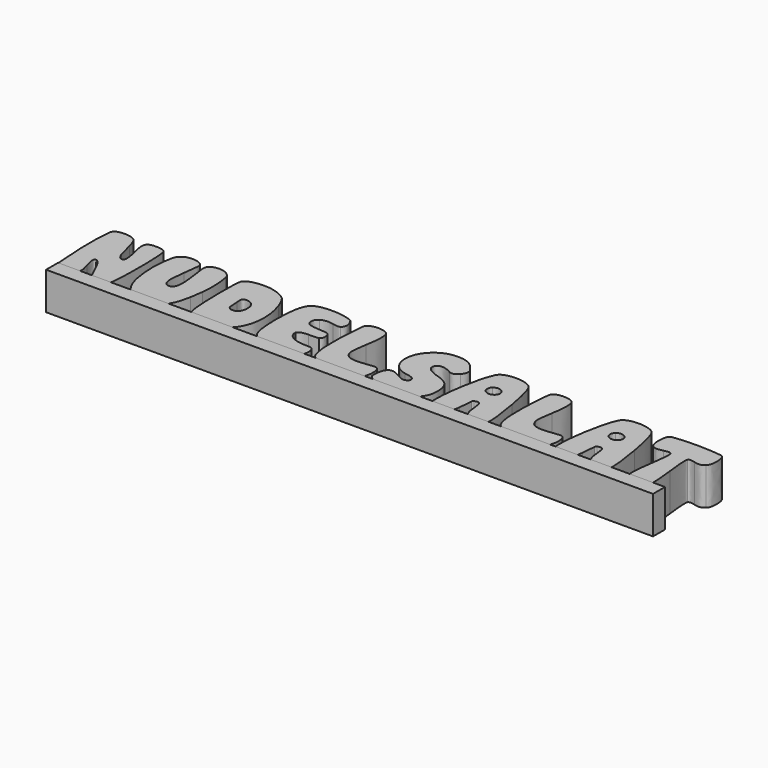
from build123d import *

# Parameters (mm, degrees)
F1_DEPTH = 10
F2_W     = 162
F2_H     = 4
F3_DEPTH = 10


# Not quite as in the source:
# - the dataset's text gives a spline's control points without its knots; the knots are read off the source's solid


with BuildPart() as f1:
    # F0 (on Top) → F1 (new body)
    with BuildSketch(Plane.XY):
        with BuildLine():
            add(Edge.make_bspline(
                [(-78.6229949402, 10.3743381), (-77.2540190734, 10.3743381), (-76.2557894812, 10.0700247503), (-75.628596004, 9.4616875221)],
                knots=[0, 0, 0, 0, 1, 1, 1, 1], degree=3))
            add(Edge.make_bspline(
                [(-81.5318144928, 8.9769327547), (-81.3989493816, 9.9081493719), (-80.4291492678, 10.3743381), (-78.6229949402, 10.3743381)],
                knots=[26, 26, 26, 26, 27, 27, 27, 27], degree=3))
            add(Edge.make_bspline(
                [(-81.3035069281, -8.7327223423), (-81.6841162725, -3.8660267327), (-81.8738407099, 0.0317393925), (-81.8738407099, 2.9597057731), (-81.8738407099, 5.3930535779), (-81.7598318478, 7.3985055723), (-81.5318144928, 8.9769327547)],
                knots=[24, 24, 24, 24, 25, 25, 25, 26, 26, 26, 26], degree=3))
            add(Edge.make_bspline(
                [(-80.1056890901, -9.8449607967), (-80.8094687718, -9.5980868234), (-81.2086445248, -9.2273405489), (-81.3035069281, -8.7327223423)],
                knots=[23, 23, 23, 23, 24, 24, 24, 24], degree=3))
            add(Edge.make_bspline(
                [(-75.6570258517, -8.8183013567), (-75.9804856602, -9.7120953163), (-76.8931362381, -10.158557166), (-78.3946870063, -10.158557166), (-79.0033140749, -10.158557166), (-79.5736482259, -10.0544117431), (-80.1056890901, -9.8449607967)],
                knots=[21, 21, 21, 21, 22, 22, 22, 23, 23, 23, 23], degree=3))
            add(Edge.make_bspline(
                [(-75.9706225903, -5.6100998048), (-75.6097397549, -6.7223382591), (-75.4287179178, -7.5447679435), (-75.4287179178, -8.0768091769), (-75.4287179178, -8.4191256037), (-75.5050139125, -8.6662897867), (-75.6570258517, -8.8183013567)],
                knots=[19, 19, 19, 19, 20, 20, 20, 21, 21, 21, 21], degree=3))
            add(Edge.make_bspline(
                [(-76.0846310832, -2.4871874267), (-76.3700881838, -2.5254803444), (-76.5125268936, -2.7537882783), (-76.5125268936, -3.1718202804), (-76.5125268936, -3.6850048955), (-76.3320854759, -4.4978613505), (-75.9706225903, -5.6100998048)],
                knots=[17, 17, 17, 17, 18, 18, 18, 19, 19, 19, 19], degree=3))
            add(Edge.make_bspline(
                [(-74.2596205065, -4.5405059374), (-74.9253967418, -3.2101135672), (-75.5334437602, -2.5254803444), (-76.0846310832, -2.4871874267)],
                knots=[16, 16, 16, 16, 17, 17, 17, 17], degree=3))
            add(Edge.make_bspline(
                [(-72.463039039, -8.2479672057), (-73.2613909142, -6.5938244481), (-73.8604443843, -5.358294112), (-74.2596205065, -4.5405059374)],
                knots=[15, 15, 15, 15, 16, 16, 16, 16], degree=3))
            add(Edge.make_bspline(
                [(-71.2367920918, -9.5882233842), (-71.9025683272, -9.2650534162), (-72.311027469, -8.8183013567), (-72.463039039, -8.2479672057)],
                knots=[14, 14, 14, 14, 15, 15, 15, 15], degree=3))
            add(Edge.make_bspline(
                [(-67.3297425778, -8.9323102188), (-67.4820447267, -9.6549461496), (-68.1666775804, -10.0161188255), (-69.3830614576, -10.0161188255), (-70.048837693, -10.0161188255), (-70.6664579408, -9.8733902751), (-71.2367920918, -9.5882233842)],
                knots=[12, 12, 12, 12, 13, 13, 13, 14, 14, 14, 14], degree=3))
            add(Edge.make_bspline(
                [(-67.3297425778, 9.0625117691), (-67.0068628195, 7.9404102449), (-66.8449878104, 5.1934657014), (-66.8449878104, 0.8208078788), (-66.8449878104, -4.179623102), (-67.0068628195, -7.4307594506), (-67.3297425778, -8.9323102188)],
                knots=[10, 10, 10, 10, 11, 11, 11, 12, 12, 12, 12], degree=3))
            add(Edge.make_bspline(
                [(-72.2634511625, 9.2049504789), (-72.0542900566, 9.7184249346), (-71.3127978768, 9.9748721372), (-70.0389746231, 9.9748721372), (-68.575136353, 9.9748721372), (-67.6720593738, 9.6705587875), (-67.3297425778, 9.0625117691)],
                knots=[8, 8, 8, 8, 9, 9, 9, 10, 10, 10, 10], degree=3))
            add(Edge.make_bspline(
                [(-71.9495645834, 5.183892472), (-72.311027469, 6.5528679696), (-72.4914688867, 7.5888104292), (-72.4914688867, 8.2925897416), (-72.4914688867, 8.729478362), (-72.4157529423, 9.0337920809), (-72.2634511625, 9.2049504789)],
                knots=[6, 6, 6, 6, 7, 7, 7, 8, 8, 8, 8], degree=3))
            add(Edge.make_bspline(
                [(-71.9211347357, 1.0775452913), (-71.5788183089, 1.1344046174), (-71.4079501206, 1.4668576051), (-71.4079501206, 2.0754846737), (-71.4079501206, 2.7786839359), (-71.588681748, 3.815206815), (-71.9495645834, 5.183892472)],
                knots=[4, 4, 4, 4, 5, 5, 5, 6, 6, 6, 6], degree=3))
            add(Edge.make_bspline(
                [(-73.489698479, 2.8454067013), (-73.03337319, 1.5715834475), (-72.5106153455, 0.9821028377), (-71.9211347357, 1.0775452913)],
                knots=[3, 3, 3, 3, 4, 4, 4, 4], degree=3))
            add(Edge.make_bspline(
                [(-74.5163575497, 6.6953066794), (-73.9651702267, 4.4711199804), (-73.6228537999, 3.1877231281), (-73.489698479, 2.8454067013)],
                knots=[2, 2, 2, 2, 3, 3, 3, 3], degree=3))
            add(Edge.make_bspline(
                [(-75.628596004, 9.4616875221), (-75.2674233281, 9.1002246365), (-74.8966770536, 8.178291039), (-74.5163575497, 6.6953066794)],
                knots=[1, 1, 1, 1, 2, 2, 2, 2], degree=3))
        make_face()
    extrude(amount=F1_DEPTH)


with BuildPart() as f1b:
    # F0 (on Top) → F1, piece 2 (new body)
    with BuildSketch(Plane.XY):
        with BuildLine():
            add(Edge.make_bspline(
                [(-57.5769146899, 8.3346542783), (-57.6912137617, 7.1072464921), (-57.8527985611, 5.7571272436), (-58.061959667, 4.2842961637)],
                knots=[0, 0, 0, 0, 1, 1, 1, 1], degree=3))
            add(Edge.make_bspline(
                [(-58.6891531442, 10.0062029747), (-57.9290945558, 9.6850637365), (-57.5484852114, 9.2316394374), (-57.5484852114, 8.6462202871), (-57.5484852114, 8.5896508015), (-57.5583482813, 8.4857955883), (-57.5769146899, 8.3346542783)],
                knots=[21, 21, 21, 21, 22, 22, 22, 23, 23, 23, 23], degree=3))
            add(Edge.make_bspline(
                [(-62.8813695491, 9.7494655623), (-62.2161729948, 10.1657570443), (-61.4459611268, 10.3743381), (-60.5713136261, 10.3743381), (-59.9061170718, 10.3743381), (-59.278633754, 10.251336428), (-58.6891531442, 10.0062029747)],
                knots=[19, 19, 19, 19, 20, 20, 20, 21, 21, 21, 21], degree=3))
            add(Edge.make_bspline(
                [(-64.1647660323, 7.8182784637), (-63.9747513852, 8.6891547146), (-63.5471457845, 9.3328838705), (-62.8813695491, 9.7494655623)],
                knots=[18, 18, 18, 18, 19, 19, 19, 19], degree=3))
            add(Edge.make_bspline(
                [(-64.136046344, -3.6838444257), (-64.5355123068, -1.8666661892), (-64.7351001833, 0.1123870565), (-64.7351001833, 2.2518646319), (-64.7351001833, 4.1261924043), (-64.5450855362, 5.9816635585), (-64.1647660323, 7.8182784637)],
                knots=[16, 16, 16, 16, 17, 17, 17, 18, 18, 18, 18], degree=3))
            add(Edge.make_bspline(
                [(-61.5979726968, -8.8809626625), (-62.7577874576, -7.896657969), (-63.6040051107, -6.1641884868), (-64.136046344, -3.6838444257)],
                knots=[15, 15, 15, 15, 16, 16, 16, 16], degree=3))
            add(Edge.make_bspline(
                [(-52.5007677645, -8.9627704271), (-52.9762395123, -9.8359676175), (-54.4783706999, -10.2725660281), (-57.0065809081, -10.2725660281), (-59.7065291953, -10.2725660281), (-61.2370898614, -9.8086982396), (-61.5979726968, -8.8809626625)],
                knots=[13, 13, 13, 13, 14, 14, 14, 15, 15, 15, 15], degree=3))
            add(Edge.make_bspline(
                [(-50.1338525153, -3.3241220601), (-50.7041866663, -6.4949009544), (-51.4932551526, -8.374450287), (-52.5007677645, -8.9627704271)],
                knots=[12, 12, 12, 12, 13, 13, 13, 13], degree=3))
            add(Edge.make_bspline(
                [(-49.6419538713, 0.057848393), (-49.7512848089, -1.0195780915), (-49.9152631002, -2.1469015451), (-50.1338525153, -3.3241220601)],
                knots=[11.5, 11.5, 11.5, 11.5, 12, 12, 12, 12], degree=3))
            add(Edge.make_bspline(
                [(-49.9342646388, 8.0390435288), (-49.6302411296, 6.6340956839), (-49.4779393499, 5.0014203246), (-49.4779393499, 3.1404370313), (-49.4779393499, 2.1628043928), (-49.5326229337, 1.1352748774), (-49.6419538713, 0.057848393)],
                knots=[10, 10, 10, 10, 11, 11, 11, 11.5, 11.5, 11.5, 11.5], degree=3))
            add(Edge.make_bspline(
                [(-51.2460909696, 9.8048745782), (-50.5428917074, 9.3868422069), (-50.1054230368, 8.7982318571), (-49.9342646388, 8.0390435288)],
                knots=[9, 9, 9, 9, 10, 10, 10, 10], degree=3))
            add(Edge.make_bspline(
                [(-55.3240083027, 9.9188830711), (-54.7919674385, 10.22232653), (-54.1549105222, 10.3743381), (-53.4134183424, 10.3743381), (-52.5962102181, 10.3743381), (-51.8735742873, 10.1843234529), (-51.2460909696, 9.8048745782)],
                knots=[7, 7, 7, 7, 8, 8, 8, 9, 9, 9, 9], degree=3))
            add(Edge.make_bspline(
                [(-56.2082290328, 8.2972316207), (-56.265088359, 8.9986899936), (-55.9706384485, 9.5391439866), (-55.3240083027, 9.9188830711)],
                knots=[6, 6, 6, 6, 7, 7, 7, 7], degree=3))
            add(Edge.make_bspline(
                [(-55.7234742655, 4.5694634238), (-56.0086411563, 6.5235682311), (-56.170226325, 7.7660606473), (-56.2082290328, 8.2972316207)],
                knots=[5, 5, 5, 5, 6, 6, 6, 6], degree=3))
            add(Edge.make_bspline(
                [(-56.892572046, -2.2307402241), (-55.865912606, -2.2690331417), (-55.3527279909, -1.3204105858), (-55.3527279909, 0.6148379725), (-55.3527279909, 1.5631703187), (-55.4766002922, 2.8810888388), (-55.7234742655, 4.5694634238)],
                knots=[3, 3, 3, 3, 4, 4, 4, 5, 5, 5, 5], degree=3))
            add(Edge.make_bspline(
                [(-58.061959667, 4.2842961637), (-58.30912385, 2.5657515802), (-58.4327059415, 1.2814848371), (-58.4327059415, 0.4317857747), (-58.4327059415, -1.305615427), (-57.9192311167, -2.1933175665), (-56.892572046, -2.2307402241)],
                knots=[1, 1, 1, 1, 2, 2, 2, 3, 3, 3, 3], degree=3))
        make_face()
    extrude(amount=F1_DEPTH)


with BuildPart() as f1c:
    # F0 (on Top) → F1, piece 3 (new body)
    with BuildSketch(Plane.XY):
        with BuildLine():
            add(Edge.make_bspline(
                [(-44.2306343957, 9.9464426588), (-43.3562767355, 10.1747502235), (-42.462482776, 10.2887590856), (-41.5498321981, 10.2887590856), (-39.1164843933, 10.2887590856), (-37.0631658826, 9.6897052463), (-35.3901665067, 8.4921779874)],
                knots=[0, 0, 0, 0, 1, 1, 1, 2, 2, 2, 2], degree=3))
            add(Edge.make_bspline(
                [(-46.3265971241, 8.591971741), (-46.1270092476, 9.1907353705), (-45.4284518645, 9.6421289398), (-44.2306343957, 9.9464426588)],
                knots=[10, 10, 10, 10, 11, 11, 11, 11], degree=3))
            add(Edge.make_bspline(
                [(-45.5996098933, -8.9894597547), (-46.2839529064, -8.019659641), (-46.6262693332, -4.0841806485), (-46.6262693332, 2.8169772228), (-46.6262693332, 6.0681132022), (-46.5264752104, 7.9929179017), (-46.3265971241, 8.591971741)],
                knots=[8, 8, 8, 8, 9, 9, 9, 10, 10, 10, 10], degree=3))
            add(Edge.make_bspline(
                [(-37.4434850174, -9.8449607967), (-38.6032997782, -10.1684206052), (-39.7915440175, -10.3297155641), (-41.0082181046, -10.3297155641), (-43.1946919361, -10.3297155641), (-44.7252526023, -9.8832537143), (-45.5996098933, -8.9894597547)],
                knots=[6, 6, 6, 6, 7, 7, 7, 8, 8, 8, 8], degree=3))
            add(Edge.make_bspline(
                [(-35.5826470597, -9.089362337), (-36.091262579, -9.3840663657), (-36.7115660669, -9.635944611), (-37.4434850174, -9.8449607967)],
                knots=[5.5, 5.5, 5.5, 5.5, 6, 6, 6, 6], degree=3))
            add(Edge.make_bspline(
                [(-34.3919369145, -8.0768091769), (-34.67710399, -8.4571284962), (-35.0740315405, -8.7946583083), (-35.5826470597, -9.089362337)],
                knots=[5, 5, 5, 5, 5.5, 5.5, 5.5, 5.5], degree=3))
            add(Edge.make_bspline(
                [(-33.393997532, 5.0130242838), (-32.671651811, 2.9782718124), (-32.3101889253, 0.9249533018), (-32.3101889253, -1.1469316174), (-32.3101889253, -3.9228860588), (-33.0043950084, -6.2329419819), (-34.3919369145, -8.0768091769)],
                knots=[3, 3, 3, 3, 4, 4, 4, 5, 5, 5, 5], degree=3))
            add(Edge.make_bspline(
                [(-35.3901665067, 8.4921779874), (-34.7058238628, 7.9975594116), (-34.040337468, 6.8380352297), (-33.393997532, 5.0130242838)],
                knots=[2, 2, 2, 2, 3, 3, 3, 3], degree=3))
        make_face()
        with BuildLine():
            add(Edge.make_bspline(
                [(-40.9226387209, -1.7456952469), (-40.7326240739, -2.2403134535), (-40.2951554032, -2.4871874267), (-39.6108123901, -2.4871874267), (-38.9647626638, -2.4871874267), (-38.4701444573, -2.2211669947), (-38.1278280305, -1.6888359207)],
                knots=[0, 0, 0, 0, 1, 1, 1, 2, 2, 2, 2], degree=3))
            add(Edge.make_bspline(
                [(-41.1506564451, 0.9632462194), (-41.1129435778, 0.5072111402), (-41.093797119, 0.1648947134), (-41.093797119, -0.0634128513), (-41.093797119, -0.9000576442), (-41.036647583, -1.460528356), (-40.9226387209, -1.7456952469)],
                knots=[6, 6, 6, 6, 7, 7, 7, 8, 8, 8, 8], degree=3))
            add(Edge.make_bspline(
                [(-40.4091642653, 2.8741263895), (-40.9417851798, 2.8741263895), (-41.2078059811, 2.5790960594), (-41.2078059811, 1.9899056593), (-41.2078059811, 1.7618879351), (-41.1889493628, 1.4195715083), (-41.1506564451, 0.9632462194)],
                knots=[4, 4, 4, 4, 5, 5, 5, 6, 6, 6, 6], degree=3))
            add(Edge.make_bspline(
                [(-38.1278280305, -1.6888359207), (-37.8426611396, -1.2325106318), (-37.6999325893, -0.6621764808), (-37.6999325893, 0.0221661631), (-37.6999325893, 1.923182894), (-38.6032997782, 2.8741263895), (-40.4091642653, 2.8741263895)],
                knots=[2, 2, 2, 2, 3, 3, 3, 4, 4, 4, 4], degree=3))
        make_face(mode=Mode.SUBTRACT)
    extrude(amount=F1_DEPTH)


with BuildPart() as f1d:
    # F0 (on Top) → F1, piece 4 (new body)
    with BuildSketch(Plane.XY):
        with BuildLine():
            add(Edge.make_bspline(
                [(-28.4890086354, 8.7773448783), (-27.7475164556, 9.7848574902), (-25.9700818162, 10.2887590856), (-23.1561246669, 10.2887590856), (-21.0842397477, 10.2887590856), (-19.2305091136, 9.9464426588), (-17.595222605, 9.2620996456)],
                knots=[0, 0, 0, 0, 1, 1, 1, 2, 2, 2, 2], degree=3))
            add(Edge.make_bspline(
                [(-28.8881847577, -7.7632124383), (-29.6111105289, -6.4705325663), (-29.9719933643, -3.8373066752), (-29.9719933643, 0.1364652349), (-29.9719933643, 4.5468355557), (-29.4776649983, 7.4272256298), (-28.4890086354, 8.7773448783)],
                knots=[23, 23, 23, 23, 24, 24, 24, 25, 25, 25, 25], degree=3))
            add(Edge.make_bspline(
                [(-16.8821599036, -9.5597935365), (-17.9088193436, -10.0352652843), (-19.5728255404, -10.2725660281), (-21.8730180243, -10.2725660281), (-25.6184823697, -10.2725660281), (-27.9569677713, -9.436211445), (-28.8881847577, -7.7632124383)],
                knots=[21, 21, 21, 21, 22, 22, 22, 23, 23, 23, 23], degree=3))
            add(Edge.make_bspline(
                [(-16.5685635343, -5.3675775008), (-15.846217444, -5.5770288165), (-15.4847545584, -6.2230785428), (-15.4847545584, -7.3068871494), (-15.4847545584, -8.371839507), (-15.9509432865, -9.1226150757), (-16.8821599036, -9.5597935365)],
                knots=[19, 19, 19, 19, 20, 20, 20, 21, 21, 21, 21], degree=3))
            add(Edge.make_bspline(
                [(-23.1276948192, -2.167498868), (-23.0328324159, -4.3963270768), (-20.8463585844, -5.4630199544), (-16.5685635343, -5.3675775008)],
                knots=[18, 18, 18, 18, 19, 19, 19, 19], degree=3))
            add(Edge.make_bspline(
                [(-20.3900332954, -1.2325106318), (-21.8158684884, -1.2325106318), (-22.7285190662, -1.5443668504), (-23.1276948192, -2.167498868)],
                knots=[17, 17, 17, 17, 18, 18, 18, 18], degree=3))
            Line((-20.3900332954, -1.2325106318), (-17.6808016194, -1.1469316174))
            add(Edge.make_bspline(
                [(-17.2316564371, 1.0987948938), (-17.1127885002, 0.827842696), (-17.0533183017, 0.497492806), (-17.0533183017, 0.1077451775), (-17.0533183017, -0.4817350631), (-17.2627696173, -0.9000576442), (-17.6808016194, -1.1469316174)],
                knots=[12.5, 12.5, 12.5, 12.5, 13, 13, 13, 14, 14, 14, 14], degree=3))
            add(Edge.make_bspline(
                [(-17.766381003, 1.7334584567), (-17.5287900494, 1.5813015972), (-17.3505243741, 1.3697470916), (-17.2316564371, 1.0987948938)],
                knots=[12, 12, 12, 12, 12.5, 12.5, 12.5, 12.5], degree=3))
            add(Edge.make_bspline(
                [(-20.4468929908, 2.0186253476), (-18.9641984717, 1.923182894), (-18.0706943527, 1.82832086), (-17.766381003, 1.7334584567)],
                knots=[11, 11, 11, 11, 12, 12, 12, 12], degree=3))
            add(Edge.make_bspline(
                [(-23.0421158048, 2.5602398104), (-22.6620865106, 2.2750725502), (-21.7970122393, 2.094341292), (-20.4468929908, 2.0186253476)],
                knots=[10, 10, 10, 10, 11, 11, 11, 11], degree=3))
            add(Edge.make_bspline(
                [(-22.7569485447, 5.4122000368), (-23.3655756133, 5.0315903231), (-23.6695991225, 4.4995494589), (-23.6695991225, 3.815206815), (-23.6695991225, 3.2065797464), (-23.4604380166, 2.7885473751), (-23.0421158048, 2.5602398104)],
                knots=[8, 8, 8, 8, 9, 9, 9, 10, 10, 10, 10], degree=3))
            add(Edge.make_bspline(
                [(-19.3491594855, 5.7115816669), (-20.0242191097, 5.8348739179), (-20.5324720052, 5.8969548042), (-20.8747884321, 5.8969548042), (-21.5974243628, 5.8969548042), (-22.2249076805, 5.735079795), (-22.7569485447, 5.4122000368)],
                knots=[6, 6, 6, 6, 7, 7, 7, 8, 8, 8, 8], degree=3))
            add(Edge.make_bspline(
                [(-17.3384851925, 5.6689374492), (-17.4719307232, 5.5734949956), (-17.6619453703, 5.5262088989), (-17.9088193436, 5.5262088989), (-18.1939862345, 5.5262088989), (-18.6743897018, 5.5877097349), (-19.3491594855, 5.7115816669)],
                knots=[4, 4, 4, 4, 5, 5, 5, 6, 6, 6, 6], degree=3))
            add(Edge.make_bspline(
                [(-17.595222605, 9.2620996456), (-16.9868857461, 8.4823145482), (-16.6825720271, 7.7408223684), (-16.6825720271, 7.0376231062), (-16.6825720271, 6.4672889552), (-16.9013067317, 6.0109636663), (-17.3384851925, 5.6689374492)],
                knots=[2, 2, 2, 2, 3, 3, 3, 4, 4, 4, 4], degree=3))
        make_face()
    extrude(amount=F1_DEPTH)


with BuildPart() as f1e:
    # F0 (on Top) → F1, piece 5 (new body)
    with BuildSketch(Plane.XY):
        with BuildLine():
            add(Edge.make_bspline(
                [(-13.7743328941, 8.74862519), (-13.451162926, 9.6992784758), (-12.4723696331, 10.1747502235), (-10.8370834938, 10.1747502235), (-9.240090272, 10.1747502235), (-8.2517237497, 9.7561378019), (-7.8711144053, 8.9197832188)],
                knots=[0, 0, 0, 0, 1, 1, 1, 2, 2, 2, 2], degree=3))
            add(Edge.make_bspline(
                [(-13.0612701927, -8.1623881913), (-13.8982048261, -7.2311715741), (-14.3162371974, -4.749957253), (-14.3162371974, -0.7193260167), (-14.3162371974, 1.923182894), (-14.1357957797, 5.0791666296), (-13.7743328941, 8.74862519)],
                knots=[14, 14, 14, 14, 15, 15, 15, 16, 16, 16, 16], degree=3))
            add(Edge.make_bspline(
                [(-0.3140433686, -9.4170649862), (-1.8350308053, -9.9116831928), (-3.5747529466, -10.158557166), (-5.5326290037, -10.158557166), (-8.9932162988, -10.158557166), (-11.5025698886, -9.493360981), (-13.0612701927, -8.1623881913)],
                knots=[12, 12, 12, 12, 13, 13, 13, 14, 14, 14, 14], degree=3))
            add(Edge.make_bspline(
                [(0.5701773615, -8.0483793292), (0.3607260459, -8.8281647959), (0.0662757661, -9.2844900848), (-0.3140433686, -9.4170649862)],
                knots=[11, 11, 11, 11, 12, 12, 12, 12], degree=3))
            add(Edge.make_bspline(
                [(-0.6560699549, -3.884592772), (0.3322965674, -3.8088771967), (0.826914774, -4.6168019321), (0.826914774, -6.3086575572), (0.826914774, -6.8604252996), (0.7413357596, -7.4400424703), (0.5701773615, -8.0483793292)],
                knots=[9, 9, 9, 9, 10, 10, 10, 11, 11, 11, 11], degree=3))
            add(Edge.make_bspline(
                [(-2.7665376323, -4.1129007059), (-1.8730338825, -3.9988918438), (-1.1695444105, -3.9228860588), (-0.6560699549, -3.884592772)],
                knots=[8, 8, 8, 8, 9, 9, 9, 9], degree=3))
            add(Edge.make_bspline(
                [(-8.4698780348, -2.3447490862), (-8.1661447353, -3.656575417), (-7.0347598222, -4.3124885824), (-5.0763037148, -4.3124885824), (-4.5822655585, -4.3124885824), (-3.812343531, -4.2460560268), (-2.7665376323, -4.1129007059)],
                knots=[6, 6, 6, 6, 7, 7, 7, 8, 8, 8, 8], degree=3))
            add(Edge.make_bspline(
                [(-8.1278518177, 2.7313978392), (-8.4513119955, 0.9063868932), (-8.6126065851, -0.4625886043), (-8.6126065851, -1.3752391821), (-8.6126065851, -1.793561394), (-8.5653204883, -2.1164411522), (-8.4698780348, -2.3447490862)],
                knots=[4, 4, 4, 4, 5, 5, 5, 6, 6, 6, 6], degree=3))
            add(Edge.make_bspline(
                [(-7.8711144053, 8.9197832188), (-7.7191028353, 8.3683056861), (-7.6430966811, 7.6836728325), (-7.6430966811, 6.8664647082), (-7.6430966811, 5.9349578813), (-7.8046818497, 4.5566989948), (-8.1278518177, 2.7313978392)],
                knots=[2, 2, 2, 2, 3, 3, 3, 4, 4, 4, 4], degree=3))
        make_face()
    extrude(amount=F1_DEPTH)


with BuildPart() as f1f:
    # F0 (on Top) → F1, piece 6 (new body)
    with BuildSketch(Plane.XY):
        with BuildLine():
            add(Edge.make_bspline(
                [(16.2262237382, 6.4101394193), (16.2262237382, 5.8206588094), (15.9645546062, 5.2311785688), (15.4420869715, 4.6422780092)],
                knots=[0, 0, 0, 0, 1, 1, 1, 1], degree=3))
            add(Edge.make_bspline(
                [(16.0266358617, 7.1803516565), (16.1592107631, 6.9520437226), (16.2262237382, 6.6953066794), (16.2262237382, 6.4101394193)],
                knots=[26, 26, 26, 26, 27, 27, 27, 27], degree=3))
            add(Edge.make_bspline(
                [(13.859308489, 9.5472669058), (14.42964264, 9.1666571921), (15.151988361, 8.3778789155), (16.0266358617, 7.1803516565)],
                knots=[25, 25, 25, 25, 26, 26, 26, 26], degree=3))
            add(Edge.make_bspline(
                [(4.5625156802, 8.2638700534), (6.1403624431, 9.7277083235), (7.9845198479, 10.4599171144), (10.0949878945, 10.4599171144), (11.6919811162, 10.4599171144), (12.9466579111, 10.1556037647), (13.859308489, 9.5472669058)],
                knots=[23, 23, 23, 23, 24, 24, 24, 25, 25, 25, 25], degree=3))
            add(Edge.make_bspline(
                [(3.2649040886, -0.5481676187), (2.5135484697, 0.402485667), (2.138450895, 1.5335803704), (2.138450895, 2.8454067013), (2.138450895, 4.936728289), (2.9460857899, 6.7425924069), (4.5625156802, 8.2638700534)],
                knots=[21, 21, 21, 21, 22, 22, 22, 23, 23, 23, 23], degree=3))
            add(Edge.make_bspline(
                [(6.3019472425, -2.3163192385), (5.0281239888, -2.0880116737), (4.0156796573, -1.4991114834), (3.2649040886, -0.5481676187)],
                knots=[20, 20, 20, 20, 21, 21, 21, 21], degree=3))
            add(Edge.make_bspline(
                [(8.2412572603, -2.8010743751), (7.9177970826, -2.6490624359), (7.2714571465, -2.4871874267), (6.3019472425, -2.3163192385)],
                knots=[19, 19, 19, 19, 20, 20, 20, 20], degree=3))
            add(Edge.make_bspline(
                [(8.9540297519, -4.1984797203), (8.9920324598, -4.0464677811), (9.0111789186, -3.9133128294), (9.0111789186, -3.7990137576), (9.0111789186, -3.3621251372), (8.7544418754, -3.0290917301), (8.2412572603, -2.8010743751)],
                knots=[17, 17, 17, 17, 18, 18, 18, 19, 19, 19, 19], degree=3))
            add(Edge.make_bspline(
                [(5.6318193379, -3.8988078804), (6.6109024713, -4.4598586426), (7.3187432433, -4.7400938139), (7.7565021237, -4.7400938139), (8.193390744, -4.7400938139), (8.5928567068, -4.5596523962), (8.9540297519, -4.1984797203)],
                knots=[15, 15, 15, 15, 16, 16, 16, 17, 17, 17, 17], degree=3))
            add(Edge.make_bspline(
                [(1.7105554538, -4.9684017478), (2.0145785938, -3.6948683346), (2.641772071, -3.0575215778), (3.5927155665, -3.0575215778), (3.9727448606, -3.0575215778), (4.6524463639, -3.3383371686), (5.6318193379, -3.8988078804)],
                knots=[13, 13, 13, 13, 14, 14, 14, 15, 15, 15, 15], degree=3))
            add(Edge.make_bspline(
                [(1.5393970558, -7.3637464756), (1.5393970558, -6.2613714604), (1.5965465917, -5.4630199544), (1.7105554538, -4.9684017478)],
                knots=[12, 12, 12, 12, 13, 13, 13, 13], degree=3))
            add(Edge.make_bspline(
                [(4.932971745, -9.816530949), (3.3548347723, -9.2650534162), (2.2240299094, -8.4475550822), (1.5393970558, -7.3637464756)],
                knots=[11, 11, 11, 11, 12, 12, 12, 12], degree=3))
            add(Edge.make_bspline(
                [(13.2602546497, -9.8449607967), (11.986431396, -10.2632830085), (10.6174555292, -10.4724441144), (9.1536176284, -10.4724441144), (7.6137735734, -10.4724441144), (6.206504789, -10.2539996196), (4.932971745, -9.816530949)],
                knots=[9, 9, 9, 9, 10, 10, 10, 11, 11, 11, 11], degree=3))
            add(Edge.make_bspline(
                [(15.6985341741, -1.0044929076), (16.2975880134, -1.8219912417), (16.5969696435, -2.9722324039), (16.5969696435, -4.454926923), (16.5969696435, -7.0408667173), (15.4847315584, -8.8374478155), (13.2602546497, -9.8449607967)],
                knots=[7, 7, 7, 7, 8, 8, 8, 9, 9, 9, 9], degree=3))
            add(Edge.make_bspline(
                [(12.6614910202, 0.8492377265), (14.0873258439, 0.4309151455), (15.0997705446, -0.1872851526), (15.6985341741, -1.0044929076)],
                knots=[6, 6, 6, 6, 7, 7, 7, 7], degree=3))
            add(Edge.make_bspline(
                [(8.8971704257, 3.3304516784), (8.9540297519, 2.4178011006), (10.2089967566, 1.5907299063), (12.6614910202, 0.8492377265)],
                knots=[5, 5, 5, 5, 6, 6, 6, 6], degree=3))
            add(Edge.make_bspline(
                [(13.1746756353, 3.9292153079), (12.1668728137, 4.537552536), (11.2826517143, 4.8418658857), (10.5225931259, 4.8418658857), (9.3627787343, 4.8418658857), (8.820874431, 4.3379646595), (8.8971704257, 3.3304516784)],
                knots=[3, 3, 3, 3, 4, 4, 4, 5, 5, 5, 5], degree=3))
            add(Edge.make_bspline(
                [(15.4420869715, 4.6422780092), (14.9187487075, 4.0525075589), (14.3626296649, 3.7580572791), (13.7737294746, 3.7580572791), (13.5642781589, 3.7580572791), (13.3646902824, 3.815206815), (13.1746756353, 3.9292153079)],
                knots=[1, 1, 1, 1, 2, 2, 2, 3, 3, 3, 3], degree=3))
        make_face()
    extrude(amount=F1_DEPTH)


with BuildPart() as f1g:
    # F0 (on Top) → F1, piece 7 (new body)
    with BuildSketch(Plane.XY):
        with BuildLine():
            add(Edge.make_bspline(
                [(21.4163795256, 8.7773448783), (21.9484203898, 9.8988663523), (23.4221217298, 10.4599171144), (25.8366132855, 10.4599171144), (26.7492638634, 10.4599171144), (27.5949014661, 10.3363350229), (28.3746865636, 10.0894610496)],
                knots=[0, 0, 0, 0, 1, 1, 1, 2, 2, 2, 2], degree=3))
            add(Edge.make_bspline(
                [(19.2774816314, 0.7352288644), (19.9049653183, 4.4041070054), (20.6180276504, 7.084909203), (21.4163795256, 8.7773448783)],
                knots=[20, 20, 20, 20, 21, 21, 21, 21], degree=3))
            add(Edge.make_bspline(
                [(18.7642970163, -9.1606177835), (18.5739925286, -8.9894597547), (18.4791301254, -8.3434096593), (18.4791301254, -7.221308135), (18.4791301254, -5.0539807622), (18.7451505574, -2.4016084123), (19.2774816314, 0.7352288644)],
                knots=[18, 18, 18, 18, 19, 19, 19, 20, 20, 20, 20], degree=3))
            add(Edge.make_bspline(
                [(23.8688737893, -9.4742145221), (23.2416803121, -10.0065455961), (22.4523219852, -10.2725660281), (21.50195854, -10.2725660281), (20.2472817451, -10.2725660281), (19.3346311673, -9.9018201228), (18.7642970163, -9.1606177835)],
                knots=[16, 16, 16, 16, 17, 17, 17, 18, 18, 18, 18], degree=3))
            add(Edge.make_bspline(
                [(24.6959449835, -7.1928782873), (24.5819364906, -8.3526930481), (24.3060526194, -9.1133316868), (23.8688737893, -9.4742145221)],
                knots=[15, 15, 15, 15, 16, 16, 16, 16], degree=3))
            add(Edge.make_bspline(
                [(25.0095417221, -3.6281455693), (24.9526823959, -4.4264970753), (24.8479569227, -5.6150315244), (24.6959449835, -7.1928782873)],
                knots=[14, 14, 14, 14, 15, 15, 15, 15], degree=3))
            add(Edge.make_bspline(
                [(25.3518581489, -3.1004560052), (25.1046943351, -3.242894715), (24.9903952633, -3.4189844634), (25.0095417221, -3.6281455693)],
                knots=[13, 13, 13, 13, 14, 14, 14, 14], degree=3))
            add(Edge.make_bspline(
                [(26.9772812184, -3.7105337534), (26.8441258974, -3.161376791), (26.5305291588, -2.8866533895), (26.036201162, -2.8866533895), (25.8267498464, -2.8866533895), (25.5987321222, -2.9577274549), (25.3518581489, -3.1004560052)],
                knots=[11, 11, 11, 11, 12, 12, 12, 13, 13, 13, 13], degree=3))
            add(Edge.make_bspline(
                [(27.1983365855, -5.4291871655), (27.1365455398, -4.9368534376), (27.0628604174, -4.363981059), (26.9772812184, -3.7105337534)],
                knots=[10.5, 10.5, 10.5, 10.5, 11, 11, 11, 11], degree=3))
            add(Edge.make_bspline(
                [(27.3480274929, -6.6646086729), (27.3100246004, -6.3333159704), (27.2601276313, -5.9215208934), (27.1983365855, -5.4291871655)],
                knots=[10, 10, 10, 10, 10.5, 10.5, 10.5, 10.5], degree=3))
            add(Edge.make_bspline(
                [(28.4318360995, -9.4486856642), (27.8423554897, -8.5018036283), (27.480892604, -7.5737778415), (27.3480274929, -6.6646086729)],
                knots=[9, 9, 9, 9, 10, 10, 10, 10], degree=3))
            add(Edge.make_bspline(
                [(32.1105776796, -10.0735585711), (31.5782466057, -10.2064236823), (31.1219213168, -10.2725660281), (30.7416018128, -10.2725660281), (29.8292414448, -10.2725660281), (29.0593197865, -9.9981328364), (28.4318360995, -9.4486856642)],
                knots=[7, 7, 7, 7, 8, 8, 8, 9, 9, 9, 9], degree=3))
            add(Edge.make_bspline(
                [(33.2799656699, -9.4469451442), (33.1465201392, -9.6938191175), (32.7566274059, -9.9024001731), (32.1105776796, -10.0735585711)],
                knots=[6, 6, 6, 6, 7, 7, 7, 7], degree=3))
            add(Edge.make_bspline(
                [(32.4813239541, 0.5208458292), (33.1845232163, -3.3905546157), (33.5364128725, -6.2477367714), (33.5364128725, -8.051280319), (33.5364128725, -8.8676181833), (33.4508334889, -9.3329362821), (33.2799656699, -9.4469451442)],
                knots=[4, 4, 4, 4, 5, 5, 5, 6, 6, 6, 6], degree=3))
            add(Edge.make_bspline(
                [(30.3995755958, 8.6937962244), (31.0647717809, 7.3840006234), (31.7586880234, 4.659683948), (32.4813239541, 0.5208458292)],
                knots=[3, 3, 3, 3, 4, 4, 4, 4], degree=3))
            add(Edge.make_bspline(
                [(28.3746865636, 10.0894610496), (29.4202022526, 9.7857277502), (30.0952618768, 9.3204096513), (30.3995755958, 8.6937962244)],
                knots=[2, 2, 2, 2, 3, 3, 3, 3], degree=3))
        make_face()
        with BuildLine():
            add(Edge.make_bspline(
                [(23.9828826514, 2.9597057731), (23.9828826514, 2.5033804842), (24.1540406802, 2.1277024901), (24.496357107, 1.8332522103)],
                knots=[0, 0, 0, 0, 1, 1, 1, 1], degree=3))
            add(Edge.make_bspline(
                [(24.496357107, 4.0861589667), (24.1540406802, 3.7911286366), (23.9828826514, 3.4160306928), (23.9828826514, 2.9597057731)],
                knots=[7, 7, 7, 7, 8, 8, 8, 8], degree=3))
            add(Edge.make_bspline(
                [(26.9062071529, 4.0861589667), (26.554027287, 4.3806088772), (26.1504998647, 4.5279793066), (25.694174945, 4.5279793066), (25.237849656, 4.5279793066), (24.8386735338, 4.3806088772), (24.496357107, 4.0861589667)],
                knots=[5, 5, 5, 5, 6, 6, 6, 7, 7, 7, 7], degree=3))
            add(Edge.make_bspline(
                [(26.9062071529, 1.8332522103), (27.2575167589, 2.1277024901), (27.4336065073, 2.5033804842), (27.4336065073, 2.9597057731), (27.4336065073, 3.4160306928), (27.2575167589, 3.7911286366), (26.9062071529, 4.0861589667)],
                knots=[3, 3, 3, 3, 4, 4, 4, 5, 5, 5, 5], degree=3))
            add(Edge.make_bspline(
                [(24.496357107, 1.8332522103), (24.8386735338, 1.5382218803), (25.237849656, 1.3911420298), (25.694174945, 1.3911420298), (26.1504998647, 1.3911420298), (26.554027287, 1.5382218803), (26.9062071529, 1.8332522103)],
                knots=[1, 1, 1, 1, 2, 2, 2, 3, 3, 3, 3], degree=3))
        make_face(mode=Mode.SUBTRACT)
    extrude(amount=F1_DEPTH)


with BuildPart() as f1h:
    # F0 (on Top) → F1, piece 8 (new body)
    with BuildSketch(Plane.XY):
        with BuildLine():
            add(Edge.make_bspline(
                [(35.7605995715, 8.74862519), (36.0837695395, 9.6992784758), (37.0625624632, 10.1747502235), (38.6978486025, 10.1747502235), (40.2948421935, 10.1747502235), (41.2832083466, 9.7561378019), (41.663817691, 8.9197832188)],
                knots=[0, 0, 0, 0, 1, 1, 1, 2, 2, 2, 2], degree=3))
            add(Edge.make_bspline(
                [(36.4736619036, -8.1623881913), (35.6367272702, -7.2311715741), (35.2186952682, -4.749957253), (35.2186952682, -0.7193260167), (35.2186952682, 1.923182894), (35.3991363166, 5.0791666296), (35.7605995715, 8.74862519)],
                knots=[14, 14, 14, 14, 15, 15, 15, 16, 16, 16, 16], degree=3))
            add(Edge.make_bspline(
                [(49.2208887277, -9.4170649862), (47.699901291, -9.9116831928), (45.9601795189, -10.158557166), (44.0023034618, -10.158557166), (40.5417161667, -10.158557166), (38.0323622077, -9.493360981), (36.4736619036, -8.1623881913)],
                knots=[12, 12, 12, 12, 13, 13, 13, 14, 14, 14, 14], degree=3))
            add(Edge.make_bspline(
                [(50.1051094578, -8.0483793292), (49.8956581422, -8.8281647959), (49.6012082316, -9.2844900848), (49.2208887277, -9.4170649862)],
                knots=[11, 11, 11, 11, 12, 12, 12, 12], degree=3))
            add(Edge.make_bspline(
                [(48.8788625106, -3.884592772), (49.8672286637, -3.8088771967), (50.3618468703, -4.6168019321), (50.3618468703, -6.3086575572), (50.3618468703, -6.8604252996), (50.2762678559, -7.4400424703), (50.1051094578, -8.0483793292)],
                knots=[9, 9, 9, 9, 10, 10, 10, 11, 11, 11, 11], degree=3))
            add(Edge.make_bspline(
                [(46.768394464, -4.1129007059), (47.6618982138, -3.9988918438), (48.3653876858, -3.9228860588), (48.8788625106, -3.884592772)],
                knots=[8, 8, 8, 8, 9, 9, 9, 9], degree=3))
            add(Edge.make_bspline(
                [(41.0650540615, -2.3447490862), (41.368787361, -3.656575417), (42.5001722741, -4.3124885824), (44.4586287507, -4.3124885824), (44.9526665378, -4.3124885824), (45.7225885653, -4.2460560268), (46.768394464, -4.1129007059)],
                knots=[6, 6, 6, 6, 7, 7, 7, 8, 8, 8, 8], degree=3))
            add(Edge.make_bspline(
                [(41.4070802786, 2.7313978392), (41.0836204701, 0.9063868932), (40.9223255112, -0.4625886043), (40.9223255112, -1.3752391821), (40.9223255112, -1.793561394), (40.969611608, -2.1164411522), (41.0650540615, -2.3447490862)],
                knots=[4, 4, 4, 4, 5, 5, 5, 6, 6, 6, 6], degree=3))
            add(Edge.make_bspline(
                [(41.663817691, 8.9197832188), (41.8158296302, 8.3683056861), (41.8918354152, 7.6836728325), (41.8918354152, 6.8664647082), (41.8918354152, 5.9349578813), (41.7302502466, 4.5566989948), (41.4070802786, 2.7313978392)],
                knots=[2, 2, 2, 2, 3, 3, 3, 4, 4, 4, 4], degree=3))
        make_face()
    extrude(amount=F1_DEPTH)


with BuildPart() as f1i:
    # F0 (on Top) → F1, piece 9 (new body)
    with BuildSketch(Plane.XY):
        with BuildLine():
            add(Edge.make_bspline(
                [(54.2398861171, 8.7773448783), (54.7719273505, 9.8988663523), (56.2456286905, 10.4599171144), (58.660119877, 10.4599171144), (59.5727704548, 10.4599171144), (60.4184084268, 10.3363350229), (61.1981935243, 10.0894610496)],
                knots=[0, 0, 0, 0, 1, 1, 1, 2, 2, 2, 2], degree=3))
            add(Edge.make_bspline(
                [(52.100988592, 0.7352288644), (52.7284719098, 4.4041070054), (53.4415346111, 7.084909203), (54.2398861171, 8.7773448783)],
                knots=[20, 20, 20, 20, 21, 21, 21, 21], degree=3))
            add(Edge.make_bspline(
                [(51.5878039769, -9.1606177835), (51.3974991201, -8.9894597547), (51.302637086, -8.3434096593), (51.302637086, -7.221308135), (51.302637086, -5.0539807622), (51.5686575181, -2.4016084123), (52.100988592, 0.7352288644)],
                knots=[18, 18, 18, 18, 19, 19, 19, 20, 20, 20, 20], degree=3))
            add(Edge.make_bspline(
                [(56.69238075, -9.4742145221), (56.0651872728, -10.0065455961), (55.2758285767, -10.2725660281), (54.3254655007, -10.2725660281), (53.0707887058, -10.2725660281), (52.158138128, -9.9018201228), (51.5878039769, -9.1606177835)],
                knots=[16, 16, 16, 16, 17, 17, 17, 18, 18, 18, 18], degree=3))
            add(Edge.make_bspline(
                [(57.5194519442, -7.1928782873), (57.4054430821, -8.3526930481), (57.1295592109, -9.1133316868), (56.69238075, -9.4742145221)],
                knots=[15, 15, 15, 15, 16, 16, 16, 16], degree=3))
            add(Edge.make_bspline(
                [(57.8330486828, -3.6281455693), (57.7761893566, -4.4264970753), (57.6714638834, -5.6150315244), (57.5194519442, -7.1928782873)],
                knots=[14, 14, 14, 14, 15, 15, 15, 15], degree=3))
            add(Edge.make_bspline(
                [(58.1753651096, -3.1004560052), (57.9282009266, -3.242894715), (57.813902224, -3.4189844634), (57.8330486828, -3.6281455693)],
                knots=[13, 13, 13, 13, 14, 14, 14, 14], degree=3))
            add(Edge.make_bspline(
                [(59.800788179, -3.7105337534), (59.6676328581, -3.161376791), (59.3540361195, -2.8866533895), (58.8597081227, -2.8866533895), (58.6502568071, -2.8866533895), (58.4222390829, -2.9577274549), (58.1753651096, -3.1004560052)],
                knots=[11, 11, 11, 11, 12, 12, 12, 13, 13, 13, 13], degree=3))
            add(Edge.make_bspline(
                [(60.0218432231, -5.4291871655), (59.9600522235, -4.9368534376), (59.8863671934, -4.363981059), (59.800788179, -3.7105337534)],
                knots=[10.5, 10.5, 10.5, 10.5, 11, 11, 11, 11], degree=3))
            add(Edge.make_bspline(
                [(60.1715340843, -6.6646086729), (60.1335311918, -6.3333159704), (60.0836342227, -5.9215208934), (60.0218432231, -5.4291871655)],
                knots=[10, 10, 10, 10, 10.5, 10.5, 10.5, 10.5], degree=3))
            add(Edge.make_bspline(
                [(61.2553430602, -9.4486856642), (60.6658624504, -8.5018036283), (60.3043995647, -7.5737778415), (60.1715340843, -6.6646086729)],
                knots=[9, 9, 9, 9, 10, 10, 10, 10], degree=3))
            add(Edge.make_bspline(
                [(64.9340846403, -10.0735585711), (64.4017535664, -10.2064236823), (63.9454282775, -10.2725660281), (63.5651087735, -10.2725660281), (62.6527484054, -10.2725660281), (61.8828263779, -9.9981328364), (61.2553430602, -9.4486856642)],
                knots=[7, 7, 7, 7, 8, 8, 8, 9, 9, 9, 9], degree=3))
            add(Edge.make_bspline(
                [(66.1034722613, -9.4469451442), (65.9700270999, -9.6938191175), (65.5801343666, -9.9024001731), (64.9340846403, -10.0735585711)],
                knots=[6, 6, 6, 6, 7, 7, 7, 7], degree=3))
            add(Edge.make_bspline(
                [(65.3048305456, 0.5208458292), (66.0080298078, -3.3905546157), (66.359919464, -6.2477367714), (66.359919464, -8.051280319), (66.359919464, -8.8676181833), (66.2743404496, -9.3329362821), (66.1034722613, -9.4469451442)],
                knots=[4, 4, 4, 4, 5, 5, 5, 6, 6, 6, 6], degree=3))
            add(Edge.make_bspline(
                [(63.2230825565, 8.6937962244), (63.8882787415, 7.3840006234), (64.5821946148, 4.659683948), (65.3048305456, 0.5208458292)],
                knots=[3, 3, 3, 3, 4, 4, 4, 4], degree=3))
            add(Edge.make_bspline(
                [(61.1981935243, 10.0894610496), (62.2437092133, 9.7857277502), (62.9187688375, 9.3204096513), (63.2230825565, 8.6937962244)],
                knots=[2, 2, 2, 2, 3, 3, 3, 3], degree=3))
        make_face()
        with BuildLine():
            add(Edge.make_bspline(
                [(56.8063892428, 2.9597057731), (56.8063892428, 2.5033804842), (56.9775476409, 2.1277024901), (57.3198640677, 1.8332522103)],
                knots=[0, 0, 0, 0, 1, 1, 1, 1], degree=3))
            add(Edge.make_bspline(
                [(57.3198640677, 4.0861589667), (56.9775476409, 3.7911286366), (56.8063892428, 3.4160306928), (56.8063892428, 2.9597057731)],
                knots=[7, 7, 7, 7, 8, 8, 8, 8], degree=3))
            add(Edge.make_bspline(
                [(59.7297141136, 4.0861589667), (59.3775342477, 4.3806088772), (58.9740068254, 4.5279793066), (58.5176815364, 4.5279793066), (58.0613562475, 4.5279793066), (57.6621804945, 4.3806088772), (57.3198640677, 4.0861589667)],
                knots=[5, 5, 5, 5, 6, 6, 6, 7, 7, 7, 7], degree=3))
            add(Edge.make_bspline(
                [(59.7297141136, 1.8332522103), (60.0810233504, 2.1277024901), (60.257113468, 2.5033804842), (60.257113468, 2.9597057731), (60.257113468, 3.4160306928), (60.0810233504, 3.7911286366), (59.7297141136, 4.0861589667)],
                knots=[3, 3, 3, 3, 4, 4, 4, 5, 5, 5, 5], degree=3))
            add(Edge.make_bspline(
                [(57.3198640677, 1.8332522103), (57.6621804945, 1.5382218803), (58.0613562475, 1.3911420298), (58.5176815364, 1.3911420298), (58.9740068254, 1.3911420298), (59.3775342477, 1.5382218803), (59.7297141136, 1.8332522103)],
                knots=[1, 1, 1, 1, 2, 2, 2, 3, 3, 3, 3], degree=3))
        make_face(mode=Mode.SUBTRACT)
    extrude(amount=F1_DEPTH)


with BuildPart() as f1j:
    # F0 (on Top) → F1, piece 10 (new body)
    with BuildSketch(Plane.XY):
        with BuildLine():
            add(Edge.make_bspline(
                [(67.4440182804, 9.9481831788), (69.0218650433, 10.2321895999), (71.2083392441, 10.3743381), (74.0031499346, 10.3743381), (76.5696530603, 10.3743381), (78.8602723148, 10.2321895999), (80.8758779581, 9.9481831788)],
                knots=[0, 0, 0, 0, 1, 1, 1, 2, 2, 2, 2], degree=3))
            add(Edge.make_bspline(
                [(67.4440182804, 4.1560725623), (66.8165349627, 4.4777922201), (66.5029382241, 5.4336674351), (66.5029382241, 7.0239884172), (66.5029382241, 8.5948727308), (66.8165349627, 9.5696041949), (67.4440182804, 9.9481831788)],
                knots=[22, 22, 22, 22, 23, 23, 23, 24, 24, 24, 24], degree=3))
            add(Edge.make_bspline(
                [(70.0676709421, 4.1003737059), (69.4587536637, 3.9480719262), (68.9931453551, 3.8720661412), (68.6702655968, 3.8720661412), (68.2139403079, 3.8720661412), (67.8049011158, 3.9666383347), (67.4440182804, 4.1560725623)],
                knots=[20, 20, 20, 20, 21, 21, 21, 22, 22, 22, 22], degree=3))
            add(Edge.make_bspline(
                [(72.0922697645, 3.9016560894), (71.9591144436, 4.1859527203), (71.72152349, 4.3283914301), (71.3794972729, 4.3283914301), (71.1128964213, 4.3283914301), (70.6757179604, 4.2523852759), (70.0676709421, 4.1003737059)],
                knots=[18, 18, 18, 18, 19, 19, 19, 20, 20, 20, 20], degree=3))
            add(Edge.make_bspline(
                [(71.6501592148, -2.118471882), (72.0209054893, 0.2629483162), (72.2062786266, 2.0514064954), (72.2062786266, 3.2469033938), (72.2062786266, 3.6263522685), (72.167985709, 3.8445065535), (72.0922697645, 3.9016560894)],
                knots=[16, 16, 16, 16, 17, 17, 17, 18, 18, 18, 18], degree=3))
            add(Edge.make_bspline(
                [(71.4079271206, -9.1626485133), (71.198475805, -8.9540674577), (71.094330382, -8.3941771653), (71.094330382, -7.4832671075), (71.094330382, -6.2880604188), (71.2797035193, -4.4996022397), (71.6501592148, -2.118471882)],
                knots=[14, 14, 14, 14, 15, 15, 15, 16, 16, 16, 16], degree=3))
            add(Edge.make_bspline(
                [(77.0544078277, -9.4219967058), (76.3129156479, -9.9891396573), (75.2578267295, -10.2725660281), (73.8888508627, -10.2725660281), (72.5770245319, -10.2725660281), (71.7502435474, -9.9029802234), (71.4079271206, -9.1626485133)],
                knots=[12, 12, 12, 12, 13, 13, 13, 14, 14, 14, 14], degree=3))
            add(Edge.make_bspline(
                [(76.9261842264, -2.192737147), (77.239780965, -4.612450632), (77.3967242545, -6.4267278788), (77.3967242545, -7.6361493067), (77.3967242545, -8.6570063979), (77.2827157617, -9.2522889873), (77.0544078277, -9.4219967058)],
                knots=[10, 10, 10, 10, 11, 11, 11, 12, 12, 12, 12], degree=3))
            add(Edge.make_bspline(
                [(76.5696530603, 4.0165352116), (76.4933570656, 3.9028165592), (76.4556441982, 3.6475294571), (76.4556441982, 3.2509648533), (76.4556441982, 2.0412532157), (76.6122976473, 0.2266857592), (76.9261842264, -2.192737147)],
                knots=[8, 8, 8, 8, 9, 9, 9, 10, 10, 10, 10], degree=3))
            add(Edge.make_bspline(
                [(78.3946640063, 4.1145884452), (77.8431864735, 4.257027155), (77.4440103513, 4.3283914301), (77.197136378, 4.3283914301), (76.9119694871, 4.3283914301), (76.7025181715, 4.224245638), (76.5696530603, 4.0165352116)],
                knots=[6, 6, 6, 6, 7, 7, 7, 8, 8, 8, 8], degree=3))
            add(Edge.make_bspline(
                [(81.0470363562, 4.581937643), (80.6855734705, 4.1276430839), (80.2199647927, 3.9007858294), (79.6496310109, 3.9007858294), (79.3644637508, 3.9007858294), (78.9458513292, 3.9718598948), (78.3946640063, 4.1145884452)],
                knots=[4, 4, 4, 4, 5, 5, 5, 6, 6, 6, 6], degree=3))
            add(Edge.make_bspline(
                [(80.8758779581, 9.9481831788), (81.5410745124, 9.6453201394), (81.8738177099, 8.7085913831), (81.8738177099, 7.1374168598), (81.8738177099, 5.717964066), (81.5982236791, 4.8659440641), (81.0470363562, 4.581937643)],
                knots=[2, 2, 2, 2, 3, 3, 3, 4, 4, 4, 4], degree=3))
        make_face()
    extrude(amount=F1_DEPTH)


with BuildPart() as f3:
    # F2 (on Top) → F3 (new body)
    with BuildSketch(Plane.XY):
        with Locations((-0.3943222165, -10.5003727153)):
            Rectangle(F2_W, F2_H)
    extrude(amount=F3_DEPTH)


solid = Compound([f1.part, f1b.part, f1c.part, f1d.part, f1e.part, f1f.part, f1g.part, f1h.part, f1i.part, f1j.part, f3.part])
